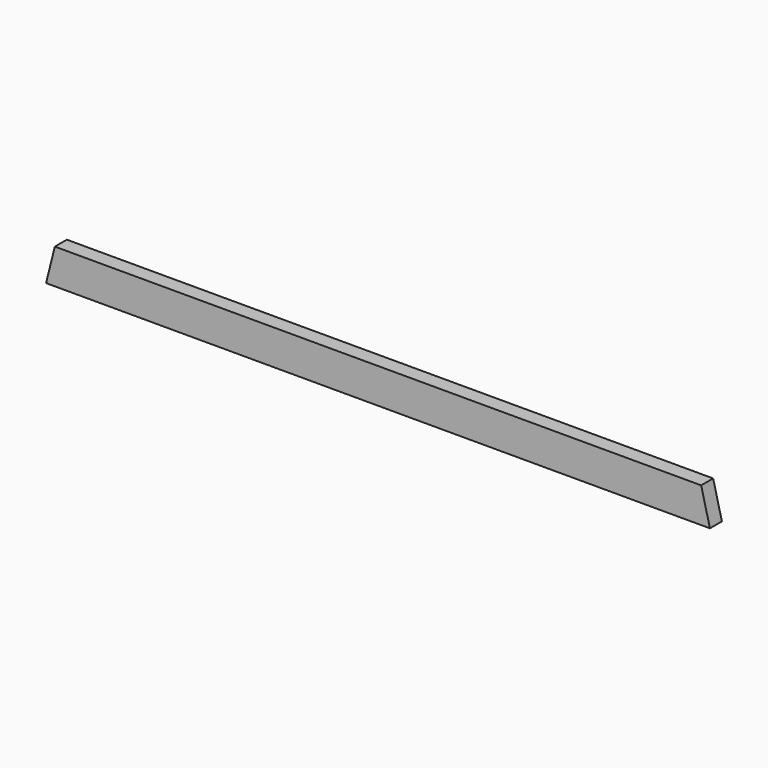
from build123d import *

# Parameters (mm, degrees)
F0_W     = 38.1
F0_H     = 88.9
F1_DEPTH = 842.9625
F2_SIZE2 = 88.89999
F2_SIZE  = 22.22499


# Not quite as in the source:
# - a fillet or chamfer is up to 0.001 mm smaller than in the source, because OpenCascade refuses the exact size


with BuildPart() as f1:
    # F0 (on Right) → F1 (new body, symmetric)
    with BuildSketch(Plane.YZ):
        Rectangle(F0_W, F0_H)
    extrude(amount=F1_DEPTH, both=True)

    # F2 (size 22.225 and 88.9 in the source; OpenCascade refuses exactly that, so slightly less here)
    f2_edges = [f1.edges().sort_by_distance(p)[0] for p in [
        (842.9625, 0, 44.45),
        (-842.9625, 0, 44.45),
    ]]
    f2_side = f1.faces().sort_by_distance((0, 0, 44.45))[0]
    chamfer(f2_edges, length=F2_SIZE, length2=F2_SIZE2, reference=f2_side)


solid = f1.part
